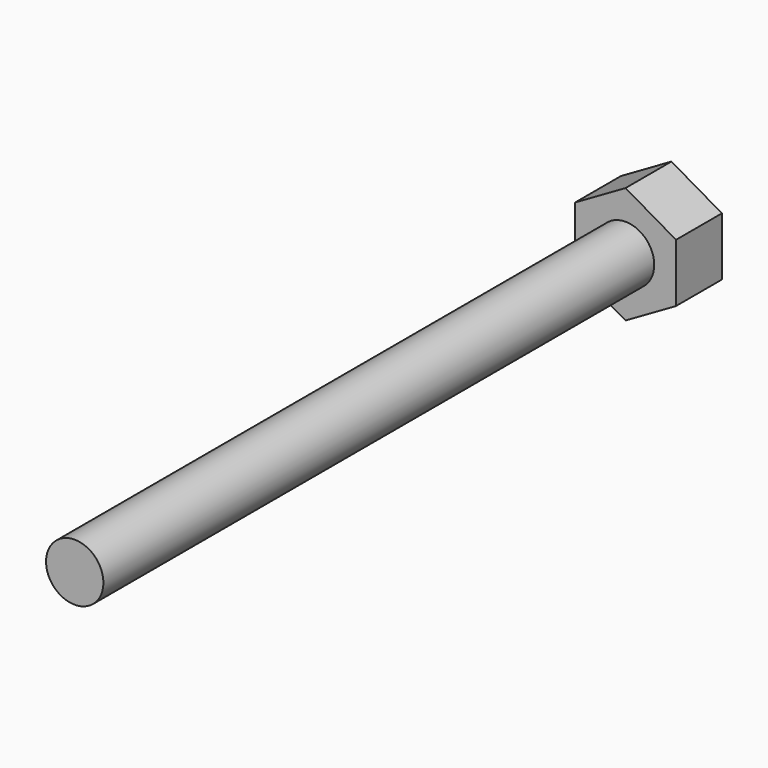
from build123d import *

# Parameters (mm, degrees)
F0_R     = 3.175
F1_DEPTH = 76.2
F2_R     = 3.175
F3_DEPTH = 6.35


with BuildPart() as f1:
    # F0 (on Front) → F1 (new body)
    with BuildSketch(Plane.XZ):
        Circle(F0_R)
    extrude(amount=F1_DEPTH)

    # F2 (on face) → F3 (join)
    with BuildSketch(Plane(origin=(0, 0, 0), x_dir=(-1, 0, 0), z_dir=(0, 1, 0))):
        Polygon((5.588, -3.2262333042), (5.588, 3.2262333042), (0, 6.4524666085), (-5.588, 3.2262333042), (-5.588, -3.2262333042), (0, -6.4524666085), align=None)
        Circle(F2_R, mode=Mode.SUBTRACT)
        Circle(F2_R)
    extrude(amount=F3_DEPTH)


solid = f1.part
